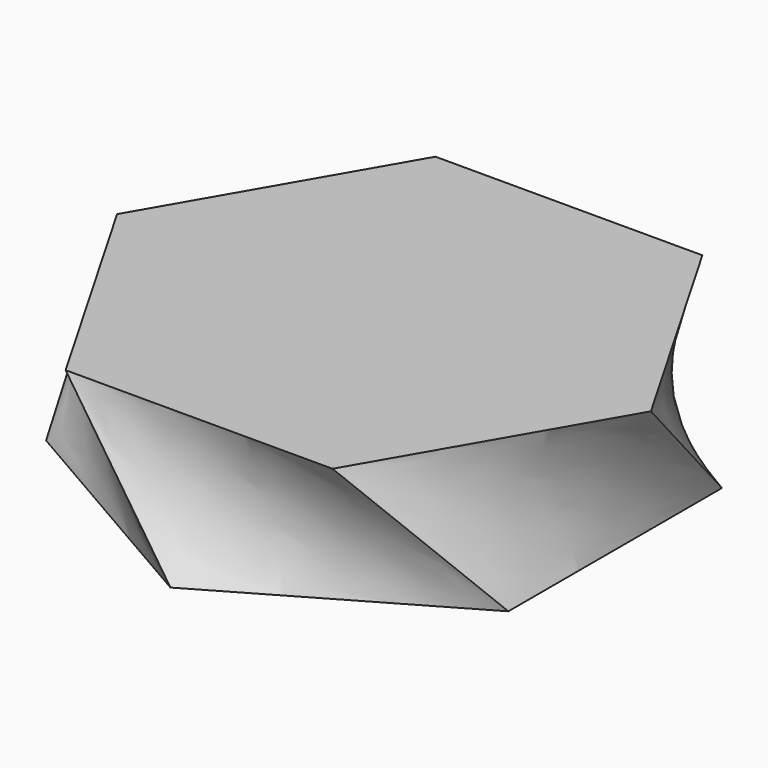
from build123d import *


with BuildPart() as f3:
    # F0 (on Top) → F3 section 0
    with BuildSketch(Plane.XY):
        Polygon((21.9970452561, -12.7), (21.9970452561, 12.7), (0, 25.4), (-21.9970452561, 12.7), (-21.9970452561, -12.7), (0, -25.4), align=None)
    # F2 (on offset) → F3 section 1
    with BuildSketch(Plane.XY.offset(12.7)):
        Polygon((-12.7, 21.9970452561), (-25.4, 0), (-12.7, -21.9970452561), (12.7, -21.9970452561), (25.4, 0), (12.7, 21.9970452561), align=None)
    loft()


solid = f3.part
